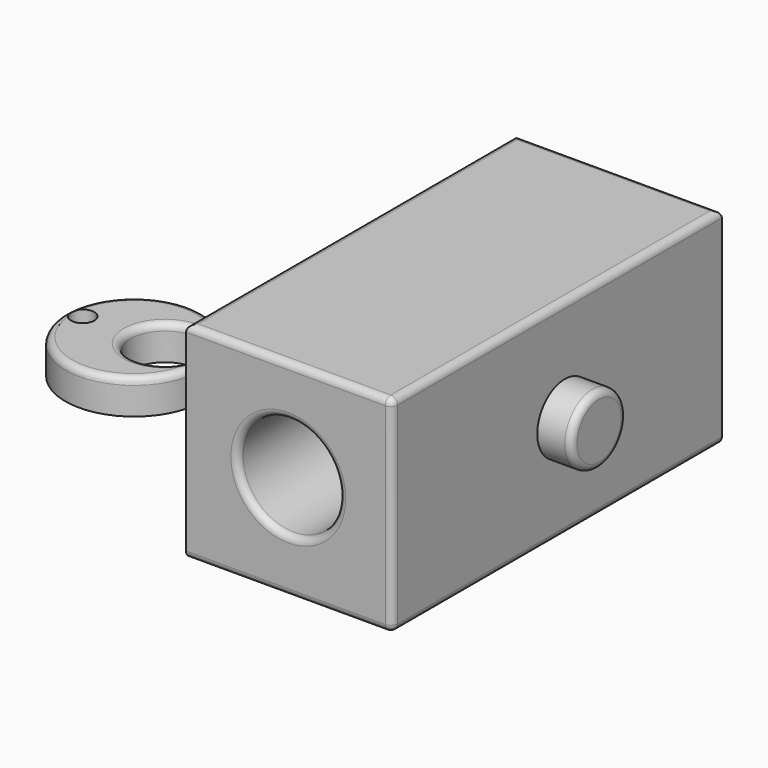
from build123d import *

# Parameters (mm, degrees)
F0_R            = 50.8
F0_R_2          = 8.6106
F1_DEPTH        = 25.4
F2_W            = 152.4
F2_H            = 304.8
F3_DEPTH        = 152.4
F5_DEPTH        = 304.8
F6_R            = 25.4
F7_DEPTH        = 25.4
F8_R            = 25.4
F9_DEPTH        = 25.4
F10_R           = 37.4754940494
F11_DEPTH       = 1270
F12_DEPTH       = 25.4
F13_DEPTH       = 25.4
F14_R           = 25.4
F15_DEPTH       = 25.4
F16_2_T1_DEPTH  = 160.0214485675
F16_2_T3_DEPTH  = 177.8048285058
F16_2_T5_DEPTH  = 330.2048285058
F16_2_T7_DEPTH  = 312.4214485675
F16_2_T9_DEPTH  = 142.2380686292
F16_2_S13_W     = 5.5895022539
F16_2_S13_H     = 5.5895022539
F16_2_T14_DEPTH = 5.589502254
F16_2_S19_W     = 5.5895022539
F16_2_S19_H     = 5.5895022539
F16_2_T20_DEPTH = 5.589502254


# Not quite as in the source:
# - a fillet or chamfer that OpenCascade refuses, or shapes differently, is made with other operations: its cross-section is extruded or revolved along the edge and cut away or added


with BuildPart() as f1:
    # F0 (on Top) → F1 (new body)
    with BuildSketch(Plane.XY):
        Circle(F0_R)
        with Locations((-39.3364430946, 1.6560875433)):
            Circle(F0_R_2, mode=Mode.SUBTRACT)
    extrude(amount=F1_DEPTH)

    # F14 (on face) → F15 (cut)
    with BuildSketch(Plane.XY.offset(25.4)):
        with Locations((19.0917998552, 4.7214571387)):
            Circle(F14_R)
    extrude(amount=-F15_DEPTH, mode=Mode.SUBTRACT)

    # F16: fillet of radius 5.08 on 2 edges, made by hand

    # F16_s1 → F16_t2 (revolve, cut)
    with BuildSketch(Plane.XZ.offset(-4.7214571387)):
        with BuildLine():
            ThreePointArc((49.5717998552, 25.4), (45.9796974068, 23.9121024484), (44.4917998552, 20.32))
            Line((44.4917998552, 20.32), (44.4917998552, 25.4))
            Line((44.4917998552, 25.4), (49.5717998552, 25.4))
        make_face()
    revolve(axis=Axis((19.0917998552, 4.7214571387, 25.4), (0, 0, 1)), mode=Mode.SUBTRACT)

    # F16_s3 → F16_t4 (revolve, cut)
    with BuildSketch(Plane.XZ):
        with BuildLine():
            ThreePointArc((50.8, 20.32), (49.3121024484, 23.9121024484), (45.72, 25.4))
            Line((45.72, 25.4), (50.8, 25.4))
            Line((50.8, 25.4), (50.8, 20.32))
        make_face()
    revolve(axis=Axis((0, 0, 25.4), (0, 0, 1)), mode=Mode.SUBTRACT)


with BuildPart() as f3:
    # F2 (on Top) → F3 (new body)
    with BuildSketch(Plane.XY):
        with Locations((242.2382127733, -7.1419849992)):
            Rectangle(F2_W, F2_H)
    extrude(amount=F3_DEPTH)

    # F4 (on face) → F5 (join)
    with BuildSketch(Plane.XZ.offset(159.5419849992)):
        with BuildLine():
            ThreePointArc((242.2382127733, 0), (296.1197494997, 22.3184632736), (318.4382127733, 76.2))
            ThreePointArc((318.4382127733, 76.2), (296.1197494997, 130.0815367264), (242.2382127733, 152.4))
            ThreePointArc((242.2382127733, 152.4), (188.3566760469, 130.0815367264), (166.0382127733, 76.2))
            ThreePointArc((166.0382127733, 76.2), (188.3566760469, 22.3184632736), (242.2382127733, 0))
        make_face()
    extrude(amount=-F5_DEPTH)

    # F6 (on face) → F7 (join)
    with BuildSketch(Plane.YZ.offset(318.4382127733)):
        with Locations((0, 76.2)):
            Circle(F6_R)
    extrude(amount=F7_DEPTH)

    # F8 (on face) → F9 (join)
    with BuildSketch(Plane(origin=(166.0382127733, 0, 0), x_dir=(0, -1, 0), z_dir=(-1, 0, 0))):
        with Locations((7.1419849992, 76.2)):
            Circle(F8_R)
    extrude(amount=F9_DEPTH)

    # F10 (on face) → F11 (cut)
    with BuildSketch(Plane.XZ.offset(159.5419849992)):
        with Locations((241.6832000017, 77.279753983)):
            Circle(F10_R)
    extrude(amount=-F11_DEPTH, mode=Mode.SUBTRACT)

    # F8 (on face) + F6 (on face) → F12 (join)
    with BuildSketch(Plane(origin=(166.0382127733, 0, 0), x_dir=(0, -1, 0), z_dir=(-1, 0, 0))):
        with Locations((7.1419849992, 76.2)):
            Circle(F8_R)
    with BuildSketch(Plane.YZ.offset(318.4382127733)):
        with Locations((0, 76.2)):
            Circle(F6_R)
    extrude(amount=-F12_DEPTH, dir=(-1, 0, 0))

    # F8 (on face) → F13 (join)
    with BuildSketch(Plane(origin=(166.0382127733, 0, 0), x_dir=(0, -1, 0), z_dir=(-1, 0, 0))):
        with Locations((7.1419849992, 76.2)):
            Circle(F8_R)
    extrude(amount=F13_DEPTH)

    # F16#2: fillet of radius 5.08 on 9 edges, made by hand

    # F16_2_s2 → F16_2_t1 (cut)
    with BuildSketch(Plane.YZ.offset(153.3357985204)):
        with BuildLine():
            ThreePointArc((-159.5423849992, 147.3190343146), (-158.0540874476, 150.9121024484), (-154.4610193138, 152.4004))
            Line((-154.4610193138, 152.4004), (-154.4610193138, 152.9085365685))
            ThreePointArc((-154.4610193138, 152.9085365685), (-157.0015021565, 152.9081365685), (-159.5419849992, 152.9081365685))
            Line((-159.5419849992, 152.9081365685), (-160.0501215677, 152.4))
            ThreePointArc((-160.0501215677, 152.4), (-160.0501215677, 149.8595171573), (-160.0505215677, 147.3190343146))
            Line((-160.0505215677, 147.3190343146), (-159.5423849992, 147.3190343146))
        make_face()
        with BuildLine():
            ThreePointArc((-159.5423849992, 5.0809656854), (-158.0540874476, 1.4878975516), (-154.4610193138, -0.0004))
            Line((-154.4610193138, -0.0004), (-154.4610193138, -0.5085365685))
            ThreePointArc((-154.4610193138, -0.5085365685), (-157.0015021565, -0.5081365685), (-159.5419849992, -0.5081365685))
            Line((-159.5419849992, -0.5081365685), (-160.0501215677, 0))
            ThreePointArc((-160.0501215677, 0), (-160.0501215677, 2.5404828427), (-160.0505215677, 5.0809656854))
            Line((-160.0505215677, 5.0809656854), (-159.5423849992, 5.0809656854))
        make_face()
    extrude(amount=F16_2_T1_DEPTH, mode=Mode.SUBTRACT)

    # F16_2_s4 → F16_2_t3 (cut)
    with BuildSketch(Plane.YZ.offset(153.3357985204)):
        with BuildLine():
            ThreePointArc((140.1770493154, 152.4004), (143.7701174492, 150.9121024484), (145.2584150008, 147.3190343146))
            Line((145.2584150008, 147.3190343146), (145.7665515694, 147.3190343146))
            ThreePointArc((145.7665515694, 147.3190343146), (145.7661515694, 149.8595171573), (145.7661515694, 152.4))
            Line((145.7661515694, 152.4), (145.2580150008, 152.9081365685))
            ThreePointArc((145.2580150008, 152.9081365685), (142.7175321581, 152.9081365685), (140.1770493154, 152.9085365685))
            Line((140.1770493154, 152.9085365685), (140.1770493154, 152.4004))
        make_face()
    extrude(amount=F16_2_T3_DEPTH, mode=Mode.SUBTRACT)

    # F16_2_s6 → F16_2_t5 (cut)
    with BuildSketch(Plane.XZ.offset(-157.9604292537)):
        with BuildLine():
            ThreePointArc((166.0378127733, 147.3190343146), (167.5261103249, 150.9121024484), (171.1191784587, 152.4004))
            Line((171.1191784587, 152.4004), (171.1191784587, 152.9085365685))
            ThreePointArc((171.1191784587, 152.9085365685), (168.578695616, 152.9081365685), (166.0382127733, 152.9081365685))
            Line((166.0382127733, 152.9081365685), (165.5300762047, 152.4))
            ThreePointArc((165.5300762047, 152.4), (165.5300762047, 149.8595171573), (165.5296762047, 147.3190343146))
            Line((165.5296762047, 147.3190343146), (166.0378127733, 147.3190343146))
        make_face()
    extrude(amount=F16_2_T5_DEPTH, mode=Mode.SUBTRACT)

    # F16_2_s8 → F16_2_t7 (cut)
    with BuildSketch(Plane.XZ.offset(-157.9604292537)):
        with BuildLine():
            ThreePointArc((318.4386127733, 147.3190343146), (316.9503152217, 150.9121024484), (313.3572470879, 152.4004))
            Line((313.3572470879, 152.4004), (313.3572470879, 152.9085365685))
            ThreePointArc((313.3572470879, 152.9085365685), (315.8977299306, 152.9081365685), (318.4382127733, 152.9081365685))
            Line((318.4382127733, 152.9081365685), (318.9463493418, 152.4))
            ThreePointArc((318.9463493418, 152.4), (318.9463493418, 149.8595171573), (318.9467493418, 147.3190343146))
            Line((318.9467493418, 147.3190343146), (318.4386127733, 147.3190343146))
        make_face()
        with BuildLine():
            ThreePointArc((313.3572470879, -0.0004), (316.9503152217, 1.4878975516), (318.4386127733, 5.0809656854))
            Line((318.4386127733, 5.0809656854), (318.9467493418, 5.0809656854))
            ThreePointArc((318.9467493418, 5.0809656854), (318.9463493418, 2.5404828427), (318.9463493418, 0))
            Line((318.9463493418, 0), (318.4382127733, -0.5081365685))
            ThreePointArc((318.4382127733, -0.5081365685), (315.8977299306, -0.5081365685), (313.3572470879, -0.5085365685))
            Line((313.3572470879, -0.5085365685), (313.3572470879, -0.0004))
        make_face()
    extrude(amount=F16_2_T7_DEPTH, mode=Mode.SUBTRACT)

    # F16_2_s10 → F16_2_t9 (cut)
    with BuildSketch(Plane.XY.offset(5.0809656854)):
        with BuildLine():
            ThreePointArc((313.3572470879, -159.5423849992), (316.9503152217, -158.0540874476), (318.4386127733, -154.4610193138))
            Line((318.4386127733, -154.4610193138), (318.9467493418, -154.4610193138))
            ThreePointArc((318.9467493418, -154.4610193138), (318.9463493418, -157.0015021565), (318.9463493418, -159.5419849992))
            Line((318.9463493418, -159.5419849992), (318.4382127733, -160.0501215677))
            ThreePointArc((318.4382127733, -160.0501215677), (315.8977299306, -160.0501215677), (313.3572470879, -160.0505215677))
            Line((313.3572470879, -160.0505215677), (313.3572470879, -159.5423849992))
        make_face()
    extrude(amount=F16_2_T9_DEPTH, mode=Mode.SUBTRACT)


with BuildPart() as f16_2_tool12:
    # F16_2_s13 → F16_2_t14 (new body)
    with BuildSketch(Plane.XZ.offset(154.4610193138)):
        with Locations((316.1519982148, 150.1137854416)):
            Rectangle(F16_2_S13_W, F16_2_S13_H)
    extrude(amount=F16_2_T14_DEPTH)

    # F16_2_s15 → F16_2_t16 (revolve, cut)
    with BuildSketch(Plane(origin=(313.3572470879, -154.4610193138, 147.3190343146), x_dir=(-0.7071067812, 0, -0.7071067812), z_dir=(-0.7071067812, 0, 0.7071067812))):
        with BuildLine():
            ThreePointArc((0, -5.0813656854), (5.0813656854, 0), (0, 5.0813656854))
            Line((0, 5.0813656854), (0, -5.0813656854))
        make_face()
    revolve(axis=Axis((313.3572470879, -154.4610193138, 147.3190343146), (0, -1, 0)), mode=Mode.SUBTRACT)


with BuildPart() as f3_1:
    add(f3.part)

    # F16_2_t11: cut F16_2_tool12
    add(f16_2_tool12.part, mode=Mode.SUBTRACT)


with BuildPart() as f16_2_tool18:
    # F16_2_s19 → F16_2_t20 (new body)
    with BuildSketch(Plane.XZ.offset(154.4610193138)):
        with Locations((316.1519982148, 2.2862145584)):
            Rectangle(F16_2_S19_W, F16_2_S19_H)
    extrude(amount=F16_2_T20_DEPTH)

    # F16_2_s21 → F16_2_t22 (revolve, cut)
    with BuildSketch(Plane(origin=(313.3572470879, -154.4610193138, 5.0809656854), x_dir=(-0.7071067812, 0, 0.7071067812), z_dir=(0.7071067812, 0, 0.7071067812))):
        with BuildLine():
            ThreePointArc((0, -5.0813656854), (5.0813656854, 0), (0, 5.0813656854))
            Line((0, 5.0813656854), (0, -5.0813656854))
        make_face()
    revolve(axis=Axis((313.3572470879, -154.4610193138, 5.0809656854), (0, -1, 0)), mode=Mode.SUBTRACT)


with BuildPart() as f3_2:
    add(f3_1.part)

    # F16_2_t17: cut F16_2_tool18
    add(f16_2_tool18.part, mode=Mode.SUBTRACT)

    # F16_2_s23 → F16_2_t24 (revolve, cut)
    with BuildSketch(Plane.XY.offset(76.2)):
        with BuildLine():
            ThreePointArc((338.7572470879, 25.4004), (342.3503152217, 23.9121024484), (343.8386127733, 20.3190343146))
            Line((343.8386127733, 20.3190343146), (344.3467493418, 20.3190343146))
            ThreePointArc((344.3467493418, 20.3190343146), (344.3463493418, 22.8595171573), (344.3463493418, 25.4))
            Line((344.3463493418, 25.4), (343.8382127733, 25.9081365685))
            ThreePointArc((343.8382127733, 25.9081365685), (341.2977299306, 25.9081365685), (338.7572470879, 25.9085365685))
            Line((338.7572470879, 25.9085365685), (338.7572470879, 25.4004))
        make_face()
    revolve(axis=Axis((343.8382127733, 0, 76.2), (1, 0, 0)), mode=Mode.SUBTRACT)

    # F16_2_s25 → F16_2_t26 (revolve, cut)
    with BuildSketch(Plane.XY.offset(77.279753983)):
        with BuildLine():
            ThreePointArc((284.2396597365, -159.5423849992), (280.6465916027, -158.0540874476), (279.1582940511, -154.4610193138))
            Line((279.1582940511, -154.4610193138), (278.6501574825, -154.4610193138))
            ThreePointArc((278.6501574825, -154.4610193138), (278.6505574825, -157.0015021565), (278.6505574825, -159.5419849992))
            Line((278.6505574825, -159.5419849992), (279.1586940511, -160.0501215677))
            ThreePointArc((279.1586940511, -160.0501215677), (281.6991768938, -160.0501215677), (284.2396597365, -160.0505215677))
            Line((284.2396597365, -160.0505215677), (284.2396597365, -159.5423849992))
        make_face()
    revolve(axis=Axis((241.6832000017, -159.5419849992, 77.279753983), (0, -1, 0)), mode=Mode.SUBTRACT)


solid = Compound([f1.part, f3_2.part])
